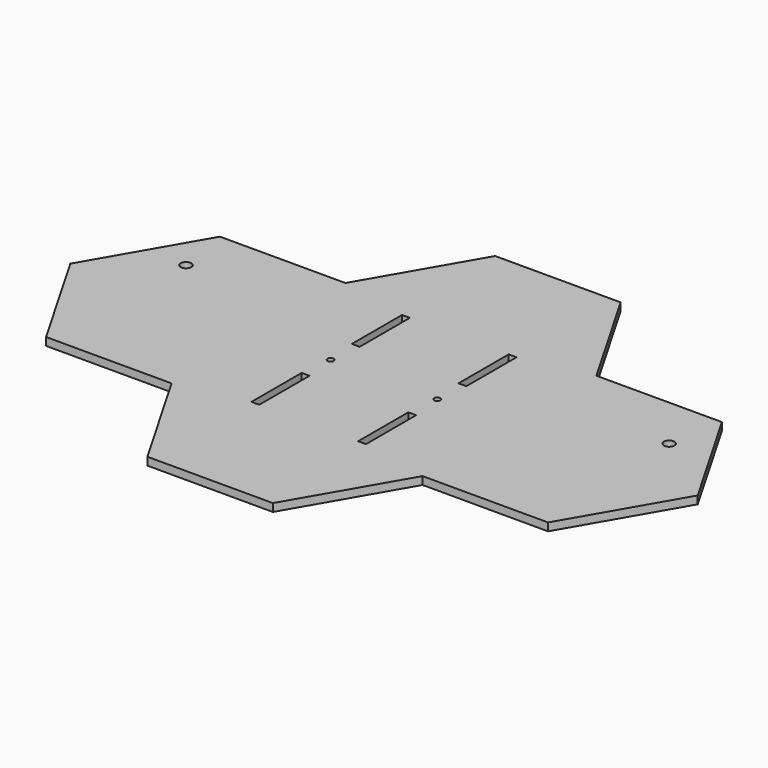
from build123d import *

# Parameters (mm, degrees)
F1_DEPTH = 3.175
F2_W     = 3.175
F2_H     = 25.4
F3_DEPTH = 7.62
F2_R     = 1.27
F4_DEPTH = 7.62
F5_R     = 2.15265
F6_DEPTH = 25.4


# Not quite as in the source:
# - a length typed as a fraction of an inch, garbled in the dataset ("3 / 203.2 mm" for 3/8 in), is restored


with BuildPart() as f1:
    # F0 (on Top) → F1 (new body)
    with BuildSketch(Plane.XY):
        Polygon((-25.4, -43.9940905122), (25.4, -43.9940905122), (50.8, 0), (101.6, 0), (127, 43.9940905122), (101.6, 87.9881810245), (50.8, 87.9881810245), (25.4, 131.9822715367), (-25.4, 131.9822715367), (-50.8, 87.9881810245), (-101.6, 87.9881810245), (-127, 43.9940905122), (-101.6, 0), (-50.8, 0), align=None)
    extrude(amount=F1_DEPTH)

    # F2 (on face) → F3 (cut)
    with BuildSketch(Plane.XY.offset(3.175)):
        with Locations((-21.59, 69.3940905122)):
            Rectangle(F2_W, F2_H)
        with Locations((21.59, 69.3940905122)):
            Rectangle(F2_W, F2_H)
        with Locations((21.59, 18.5940905122)):
            Rectangle(F2_W, F2_H)
        with Locations((-21.59, 18.5940905122)):
            Rectangle(F2_W, F2_H)
    extrude(amount=-F3_DEPTH, mode=Mode.SUBTRACT)

    # F2 (on face) → F4 (cut)
    with BuildSketch(Plane.XY.offset(3.175)):
        with Locations((-21.59, 43.9940905122)):
            Circle(F2_R)
        with Locations((21.59, 43.9940905122)):
            Circle(F2_R)
    extrude(amount=-F4_DEPTH, mode=Mode.SUBTRACT)

    # F5 (on face) → F6 (cut)
    with BuildSketch(Plane.XY.offset(3.175)):
        with Locations((97.79, 66.0370998967)):
            Circle(F5_R)
        with Locations((-97.79, 66.0370998967)):
            Circle(F5_R)
    extrude(amount=-F6_DEPTH, mode=Mode.SUBTRACT)


solid = f1.part
